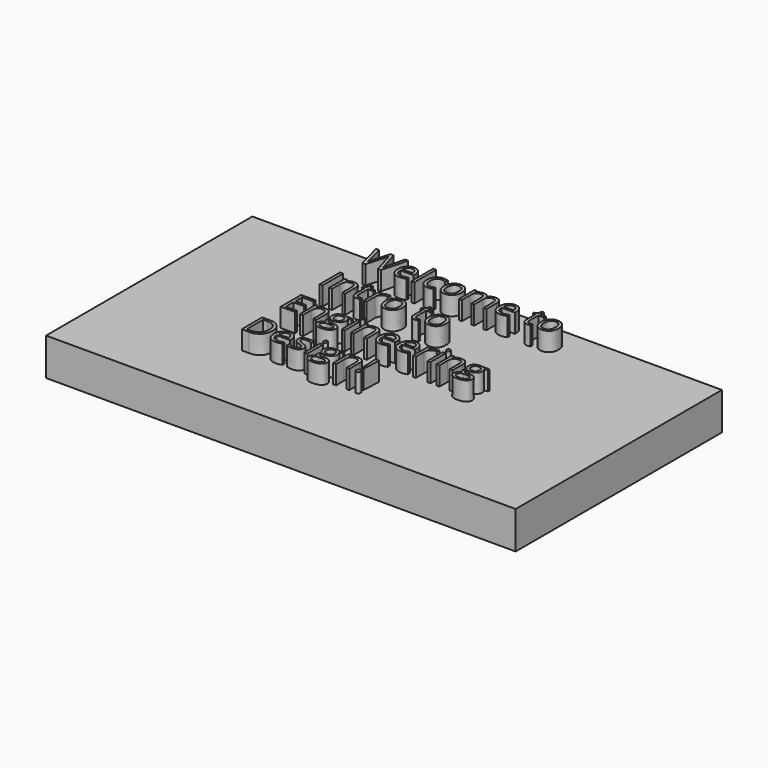
from build123d import *

# Parameters (mm, degrees)
F0_W         = 159.3459844589
F0_H         = 87.4910950661
F1_DEPTH     = 12.7
F2_TEXT_SIZE = 12.1467177653
F3_DEPTH     = 6.35


# Not quite as in the source:
# - Text() gives the source's letters only with a copy of the font that has no kerning and outlines rounded to 1/6400 em; it was checked with that copy


with BuildPart() as f1:
    # F0 (on Top) → F1 (new body)
    with BuildSketch(Plane.XY):
        Rectangle(F0_W, F0_H)
    extrude(amount=F1_DEPTH)

    # F2 (on face) → F3 (join)
    with BuildSketch(Plane.XY.offset(12.7)):
        with Locations((-35.0264962763, 31.5190888941)):
            Text('Welcome to', F2_TEXT_SIZE, font='Open Sans', text_align=(TextAlign.LEFT, TextAlign.BOTTOM))
        with Locations((-35.0264962763, 14.9995527334)):
            Text('Intro to', F2_TEXT_SIZE, font='Open Sans', text_align=(TextAlign.LEFT, TextAlign.BOTTOM))
        with Locations((-35.0264962763, -1.5199834274)):
            Text('Engineering', F2_TEXT_SIZE, font='Open Sans', text_align=(TextAlign.LEFT, TextAlign.BOTTOM))
        with Locations((-35.0264962763, -18.0395195882)):
            Text('Design!', F2_TEXT_SIZE, font='Open Sans', text_align=(TextAlign.LEFT, TextAlign.BOTTOM))
    extrude(amount=F3_DEPTH)


solid = f1.part
